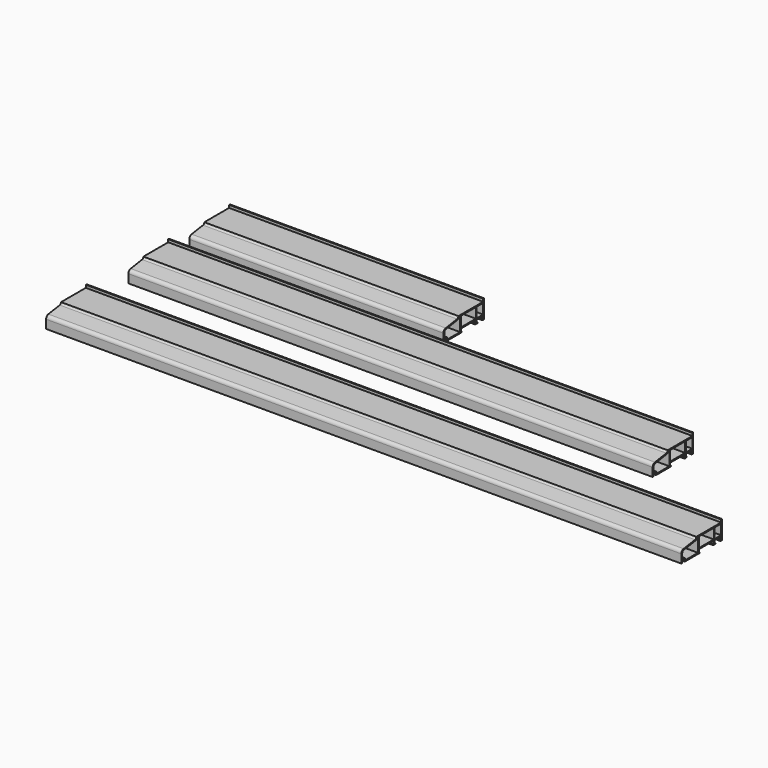
from build123d import *

# Parameters (mm, degrees)
F0_W     = 35
F0_H     = 19
F0_W_2   = 15
F1_DEPTH = 1190
F2_W     = 35
F2_H     = 19
F2_W_2   = 15
F3_DEPTH = 982
F4_W     = 35
F4_H     = 19
F4_W_2   = 15
F5_DEPTH = 434


# Not quite as in the source:
# - a pattern or mirror of a feature is missing from the dataset's text; its kind, count and spacing are read off the source's solid


with BuildPart() as f1:
    # F0 (on Right) → F1 (new body)
    with BuildSketch(Plane.YZ):
        with BuildLine():
            Line((-3.5, 0), (0, 0))
            Line((0, 0), (0, 35))
            Line((0, 35), (-2, 35))
            Line((-2, 35), (-2, 30))
            Line((-2, 30), (-60, 30))
            ThreePointArc((-60, 30), (-60.7744734264, 27.5866917079), (-62.9731507952, 26.3258650629))
            Line((-62.9731507952, 26.3258650629), (-89.6050068217, 22.2771548948))
            ThreePointArc((-89.6050068217, 22.2771548948), (-93.4659245337, 20.1384968577), (-95, 16))
            Line((-95, 16), (-95, 0))
            Line((-95, 0), (-93, 0))
            Line((-93, 0), (-93, 4))
            Line((-93, 4), (-88.5632947253, 4.5661950108))
            ThreePointArc((-88.5632947253, 4.5661950108), (-88.1695816006, 4.4454822277), (-88, 4.0702174128))
            Line((-88, 4.0702174128), (-88, 1.5))
            ThreePointArc((-88, 1.5), (-87.5606601718, 0.4393398282), (-86.5, 0))
            Line((-86.5, 0), (-52.5, 0))
            Line((-52.5, 0), (-52.5, 2))
            Line((-52.5, 2), (-54, 2))
            Line((-54, 2), (-54, 7))
            Line((-54, 7), (-19, 7))
            Line((-19, 7), (-19, 2))
            Line((-19, 2), (-20.5, 2))
            Line((-20.5, 2), (-20.5, 0))
            Line((-20.5, 0), (-15.5, 0))
            Line((-15.5, 0), (-15.5, 2))
            Line((-15.5, 2), (-17, 2))
            Line((-17, 2), (-17, 7))
            Line((-17, 7), (-2, 7))
            Line((-2, 7), (-2, 2))
            Line((-2, 2), (-3.5, 2))
            Line((-3.5, 2), (-3.5, 0))
        make_face()
        with BuildLine():
            Line((-89.3044104462, 20.2998734735), (-62.6725544196, 24.3485836416))
            ThreePointArc((-62.6725544196, 24.3485836416), (-59.9737363817, 25.5634116164), (-58.2937176737, 28))
            Line((-58.2937176737, 28), (-56, 28))
            Line((-56, 28), (-56, 2))
            Line((-56, 2), (-86, 2))
            Line((-86, 2), (-86, 4.0702174128))
            ThreePointArc((-86, 4.0702174128), (-86.8479080029, 5.9465414874), (-88.8164736264, 6.550105403))
            Line((-88.8164736264, 6.550105403), (-93, 6.0162200953))
            Line((-93, 6.0162200953), (-93, 16))
            ThreePointArc((-93, 16), (-91.9491528384, 18.8348850963), (-89.3044104462, 20.2998734735))
        make_face(mode=Mode.SUBTRACT)
        with Locations((-36.5, 18.5)):
            Rectangle(F0_W, F0_H, mode=Mode.SUBTRACT)
        with Locations((-9.5, 18.5)):
            Rectangle(F0_W_2, F0_H, mode=Mode.SUBTRACT)
    extrude(amount=F1_DEPTH)


with BuildPart() as f3:
    # F2 (on Right) → F3 (new body)
    with BuildSketch(Plane.YZ):
        with BuildLine():
            Line((189.3476232214, -3.2963262814), (192.8476232214, -3.2963262814))
            Line((192.8476232214, -3.2963262814), (192.8476232214, 31.7036737186))
            Line((192.8476232214, 31.7036737186), (190.8476232214, 31.7036737186))
            Line((190.8476232214, 31.7036737186), (190.8476232214, 26.7036737186))
            Line((190.8476232214, 26.7036737186), (132.8476232214, 26.7036737186))
            ThreePointArc((132.8476232214, 26.7036737186), (132.073149795, 24.2903654266), (129.8744724262, 23.0295387816))
            Line((129.8744724262, 23.0295387816), (103.2426163997, 18.9808286134))
            ThreePointArc((103.2426163997, 18.9808286134), (99.3816986877, 16.8421705764), (97.8476232214, 12.7036737186))
            Line((97.8476232214, 12.7036737186), (97.8476232214, -3.2963262814))
            Line((97.8476232214, -3.2963262814), (99.8476232214, -3.2963262814))
            Line((99.8476232214, -3.2963262814), (99.8476232214, 0.7036737186))
            Line((99.8476232214, 0.7036737186), (104.2843284961, 1.2698687295))
            ThreePointArc((104.2843284961, 1.2698687295), (104.6780416208, 1.1491559464), (104.8476232214, 0.7738911315))
            Line((104.8476232214, 0.7738911315), (104.8476232214, -1.7963262814))
            ThreePointArc((104.8476232214, -1.7963262814), (105.2869630496, -2.8569864531), (106.3476232214, -3.2963262814))
            Line((106.3476232214, -3.2963262814), (140.3476232214, -3.2963262814))
            Line((140.3476232214, -3.2963262814), (140.3476232214, -1.2963262814))
            Line((140.3476232214, -1.2963262814), (138.8476232214, -1.2963262814))
            Line((138.8476232214, -1.2963262814), (138.8476232214, 3.7036737186))
            Line((138.8476232214, 3.7036737186), (173.8476232214, 3.7036737186))
            Line((173.8476232214, 3.7036737186), (173.8476232214, -1.2963262814))
            Line((173.8476232214, -1.2963262814), (172.3476232214, -1.2963262814))
            Line((172.3476232214, -1.2963262814), (172.3476232214, -3.2963262814))
            Line((172.3476232214, -3.2963262814), (177.3476232214, -3.2963262814))
            Line((177.3476232214, -3.2963262814), (177.3476232214, -1.2963262814))
            Line((177.3476232214, -1.2963262814), (175.8476232214, -1.2963262814))
            Line((175.8476232214, -1.2963262814), (175.8476232214, 3.7036737186))
            Line((175.8476232214, 3.7036737186), (190.8476232214, 3.7036737186))
            Line((190.8476232214, 3.7036737186), (190.8476232214, -1.2963262814))
            Line((190.8476232214, -1.2963262814), (189.3476232214, -1.2963262814))
            Line((189.3476232214, -1.2963262814), (189.3476232214, -3.2963262814))
        make_face()
        with BuildLine():
            Line((103.5432127752, 17.0035471921), (130.1750688018, 21.0522573603))
            ThreePointArc((130.1750688018, 21.0522573603), (132.8738868397, 22.2670853351), (134.5539055477, 24.7036737186))
            Line((134.5539055477, 24.7036737186), (136.8476232214, 24.7036737186))
            Line((136.8476232214, 24.7036737186), (136.8476232214, -1.2963262814))
            Line((136.8476232214, -1.2963262814), (106.8476232214, -1.2963262814))
            Line((106.8476232214, -1.2963262814), (106.8476232214, 0.7738911315))
            ThreePointArc((106.8476232214, 0.7738911315), (105.9997152185, 2.6502152061), (104.031149595, 3.2537791216))
            Line((104.031149595, 3.2537791216), (99.8476232214, 2.719893814))
            Line((99.8476232214, 2.719893814), (99.8476232214, 12.7036737186))
            ThreePointArc((99.8476232214, 12.7036737186), (100.898470383, 15.538558815), (103.5432127752, 17.0035471921))
        make_face(mode=Mode.SUBTRACT)
        with Locations((156.3476232214, 15.2036737186)):
            Rectangle(F2_W, F2_H, mode=Mode.SUBTRACT)
        with Locations((183.3476232214, 15.2036737186)):
            Rectangle(F2_W_2, F2_H, mode=Mode.SUBTRACT)
    extrude(amount=F3_DEPTH)


with BuildPart() as f5:
    # F4 (on Right) → F5 (new body)
    with BuildSketch(Plane.YZ):
        with BuildLine():
            Line((331.9227610042, -4.5522762405), (335.4227610042, -4.5522762405))
            Line((335.4227610042, -4.5522762405), (335.4227610042, 30.4477237595))
            Line((335.4227610042, 30.4477237595), (333.4227610042, 30.4477237595))
            Line((333.4227610042, 30.4477237595), (333.4227610042, 25.4477237595))
            Line((333.4227610042, 25.4477237595), (275.4227610042, 25.4477237595))
            ThreePointArc((275.4227610042, 25.4477237595), (274.6482875779, 23.0344154674), (272.4496102091, 21.7735888224))
            Line((272.4496102091, 21.7735888224), (245.8177541825, 17.7248786542))
            ThreePointArc((245.8177541825, 17.7248786542), (241.9568364705, 15.5862206172), (240.4227610042, 11.4477237595))
            Line((240.4227610042, 11.4477237595), (240.4227610042, -4.5522762405))
            Line((240.4227610042, -4.5522762405), (242.4227610042, -4.5522762405))
            Line((242.4227610042, -4.5522762405), (242.4227610042, -0.5522762405))
            Line((242.4227610042, -0.5522762405), (246.859466279, 0.0139187703))
            ThreePointArc((246.859466279, 0.0139187703), (247.2531794037, -0.1067940128), (247.4227610042, -0.4820588277))
            Line((247.4227610042, -0.4820588277), (247.4227610042, -3.0522762405))
            ThreePointArc((247.4227610042, -3.0522762405), (247.8621008325, -4.1129364123), (248.9227610042, -4.5522762405))
            Line((248.9227610042, -4.5522762405), (282.9227610042, -4.5522762405))
            Line((282.9227610042, -4.5522762405), (282.9227610042, -2.5522762405))
            Line((282.9227610042, -2.5522762405), (281.4227610042, -2.5522762405))
            Line((281.4227610042, -2.5522762405), (281.4227610042, 2.4477237595))
            Line((281.4227610042, 2.4477237595), (316.4227610042, 2.4477237595))
            Line((316.4227610042, 2.4477237595), (316.4227610042, -2.5522762405))
            Line((316.4227610042, -2.5522762405), (314.9227610042, -2.5522762405))
            Line((314.9227610042, -2.5522762405), (314.9227610042, -4.5522762405))
            Line((314.9227610042, -4.5522762405), (319.9227610042, -4.5522762405))
            Line((319.9227610042, -4.5522762405), (319.9227610042, -2.5522762405))
            Line((319.9227610042, -2.5522762405), (318.4227610042, -2.5522762405))
            Line((318.4227610042, -2.5522762405), (318.4227610042, 2.4477237595))
            Line((318.4227610042, 2.4477237595), (333.4227610042, 2.4477237595))
            Line((333.4227610042, 2.4477237595), (333.4227610042, -2.5522762405))
            Line((333.4227610042, -2.5522762405), (331.9227610042, -2.5522762405))
            Line((331.9227610042, -2.5522762405), (331.9227610042, -4.5522762405))
        make_face()
        with BuildLine():
            Line((246.1183505581, 15.7475972329), (272.7502065846, 19.7963074011))
            ThreePointArc((272.7502065846, 19.7963074011), (275.4490246225, 21.0111353759), (277.1290433305, 23.4477237595))
            Line((277.1290433305, 23.4477237595), (279.4227610042, 23.4477237595))
            Line((279.4227610042, 23.4477237595), (279.4227610042, -2.5522762405))
            Line((279.4227610042, -2.5522762405), (249.4227610042, -2.5522762405))
            Line((249.4227610042, -2.5522762405), (249.4227610042, -0.4820588277))
            ThreePointArc((249.4227610042, -0.4820588277), (248.5748530014, 1.3942652469), (246.6062873779, 1.9978291625))
            Line((246.6062873779, 1.9978291625), (242.4227610042, 1.4639438548))
            Line((242.4227610042, 1.4639438548), (242.4227610042, 11.4477237595))
            ThreePointArc((242.4227610042, 11.4477237595), (243.4736081658, 14.2826088558), (246.1183505581, 15.7475972329))
        make_face(mode=Mode.SUBTRACT)
        with Locations((298.9227610042, 13.9477237595)):
            Rectangle(F4_W, F4_H, mode=Mode.SUBTRACT)
        with Locations((325.9227610042, 13.9477237595)):
            Rectangle(F4_W_2, F4_H, mode=Mode.SUBTRACT)
    extrude(amount=F5_DEPTH)

    # F5_copies: F5 across plane


with BuildPart() as f5_1:
    add(f5.part)
    add(f5.part.mirror(Plane(origin=(238, 0, 0), x_dir=(0, 0, 1), z_dir=(1, 0, 0))))


solid = Compound([f1.part, f3.part, f5_1.part])
